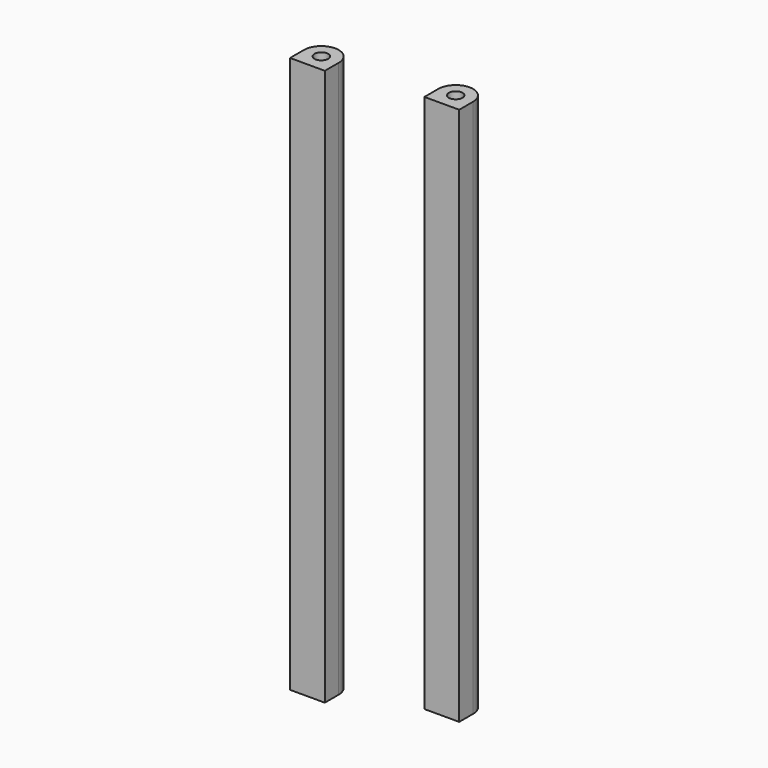
from build123d import *

# Parameters (mm, degrees)
F0_W           = 8
F0_H           = 8
F1_DEPTH       = 128
F2_DEPTH       = 124
F5_D           = 3.15
F5_DEPTH       = 15
F5_TIP         = 0.946355475
F5_2_D         = 3.15
F5_2_DEPTH     = 15
F5_2_TIP       = 0.946355475
F5_ON_F3_D     = 3.15
F5_ON_F3_DEPTH = 15
F5_ON_F3_TIP   = 0.946355475
F5_ON_F4_D     = 3.15
F5_ON_F4_DEPTH = 15
F5_ON_F4_TIP   = 0.946355475
F6_R           = 3.99999
F6_2_R         = 3.99999


# Not quite as in the source:
# - a fillet or chamfer is up to 0.001 mm smaller than in the source, because OpenCascade refuses the exact size


with BuildPart() as f1:
    # F0 (on Top) → F1 (new body)
    with BuildSketch(Plane.XY):
        with Locations((0.2846295983, -12.3607183769)):
            Rectangle(F0_W, F0_H)
    extrude(amount=-F1_DEPTH)

    # F5
    with Locations(Plane.XY):
        with Locations((0.2846295983, -12.3607183769), (28.6077857018, -9.1167669743)):
            Hole(F5_D / 2, depth=F5_DEPTH)
            with Locations((0, 0, -(F5_DEPTH + F5_TIP / 2))):  # 118° drill point
                Cone(0, F5_D / 2, F5_TIP, mode=Mode.SUBTRACT)

    # F5 on F3
    with Locations(Plane(origin=(0, 0, -128), x_dir=(1, 0, 0), z_dir=(0, 0, -1))):
        with Locations((0.2846295983, 12.3607183769)):
            Hole(F5_ON_F3_D / 2, depth=F5_ON_F3_DEPTH)
            with Locations((0, 0, -(F5_ON_F3_DEPTH + F5_ON_F3_TIP / 2))):  # 118° drill point
                Cone(0, F5_ON_F3_D / 2, F5_ON_F3_TIP, mode=Mode.SUBTRACT)

    # F6 (radius 4 in the source; OpenCascade refuses exactly that, so slightly less here)
    f6_edges = [f1.edges().sort_by_distance(p)[0] for p in [
        (-3.71537, -8.360718, -64),
        (4.28463, -8.360718, -64),
    ]]
    fillet(f6_edges, radius=F6_R)


with BuildPart() as f2:
    # F0 (on Top) → F2 (new body)
    with BuildSketch(Plane.XY):
        with Locations((28.6077857018, -9.1167669743)):
            Rectangle(F0_W, F0_H)
    extrude(amount=-F2_DEPTH)

    # F5#2
    with Locations(Plane.XY):
        with Locations((0.2846295983, -12.3607183769), (28.6077857018, -9.1167669743)):
            Hole(F5_2_D / 2, depth=F5_2_DEPTH)
            with Locations((0, 0, -(F5_2_DEPTH + F5_2_TIP / 2))):  # 118° drill point
                Cone(0, F5_2_D / 2, F5_2_TIP, mode=Mode.SUBTRACT)

    # F5 on F4
    with Locations(Plane(origin=(0, 0, -124), x_dir=(1, 0, 0), z_dir=(0, 0, -1))):
        with Locations((28.6077857018, 9.1167669743)):
            Hole(F5_ON_F4_D / 2, depth=F5_ON_F4_DEPTH)
            with Locations((0, 0, -(F5_ON_F4_DEPTH + F5_ON_F4_TIP / 2))):  # 118° drill point
                Cone(0, F5_ON_F4_D / 2, F5_ON_F4_TIP, mode=Mode.SUBTRACT)

    # F6#2 (radius 4 in the source; OpenCascade refuses exactly that, so slightly less here)
    f6_2_edges = [f2.edges().sort_by_distance(p)[0] for p in [
        (24.607786, -5.116767, -62),
        (32.607786, -5.116767, -62),
    ]]
    fillet(f6_2_edges, radius=F6_2_R)


solid = Compound([f1.part, f2.part])
